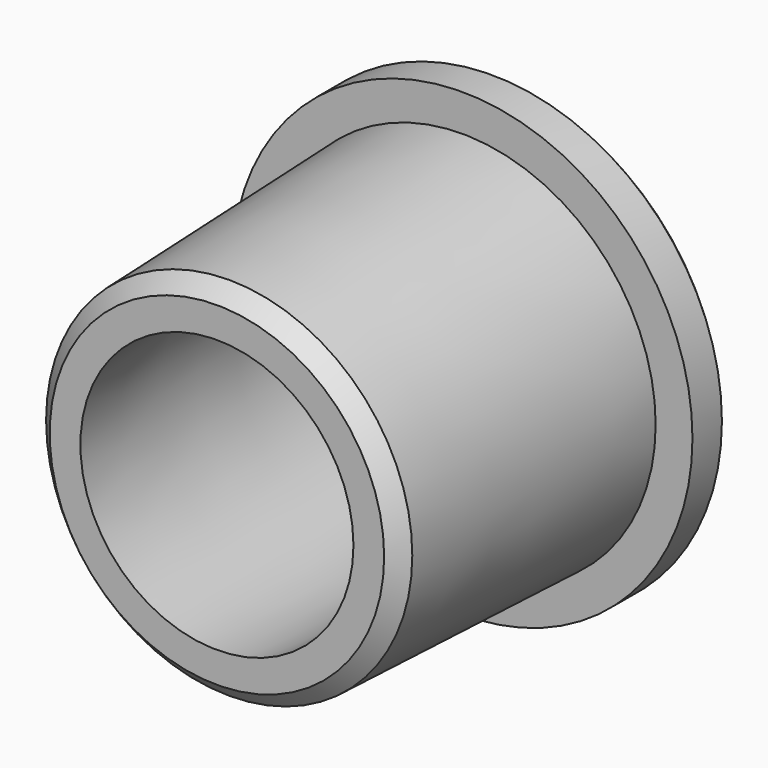
from build123d import *

# Parameters (mm, degrees)
F0_R      = 6.3
F1_DEPTH  = 10
F1_TAPER  = 2
F0_R_2    = 7.5
F1_FACE_R = 6.3
F2_DEPTH  = 1.5
F3_SIZE   = 0.3
F4_T      = -1.5


# Not quite as in the source:
# - a fillet or chamfer that OpenCascade refuses, or shapes differently, is made with other operations: its cross-section is extruded or revolved along the edge and cut away or added


with BuildPart() as f1:
    # F0 (on Front) → F1 (new body)
    with BuildSketch(Plane.XZ):
        Circle(F0_R)
    extrude(amount=F1_DEPTH, taper=F1_TAPER)

    # F0 (on Front) + F1_face (on face) → F2 (join)
    with BuildSketch(Plane.XZ):
        Circle(F0_R_2)
        Circle(F0_R, mode=Mode.SUBTRACT)
    with BuildSketch(Plane(origin=(0, 0, 0), x_dir=(1, 0, 0), z_dir=(0, 1, 0))):
        Circle(F1_FACE_R)
    extrude(amount=-F2_DEPTH, dir=(0, -1, 0))

    # F3
    f3_edges = [f1.edges().sort_by_distance(p)[0] for p in [
        (-7.5, 1.5, 0),
    ]]
    chamfer(f3_edges, length=F3_SIZE)

    # F4
    f4_openings = [f1.faces().sort_by_distance(p)[0] for p in [
        (0, -10, 0),
    ]]
    offset(amount=F4_T, openings=f4_openings, kind=Kind.INTERSECTION)

    # F5: chamfer of 0.5 on 1 edges, made by hand

    # F5_s1 → F5_t2 (revolve, cut)
    with BuildSketch(Plane.XY):
        Polygon((5.9682420534, -9.5003045865), (5.4507923051, -10), (5.9507923051, -10), align=None)
    revolve(axis=Axis((0, -10, 0), (0, 1, 0)), mode=Mode.SUBTRACT)


solid = f1.part
